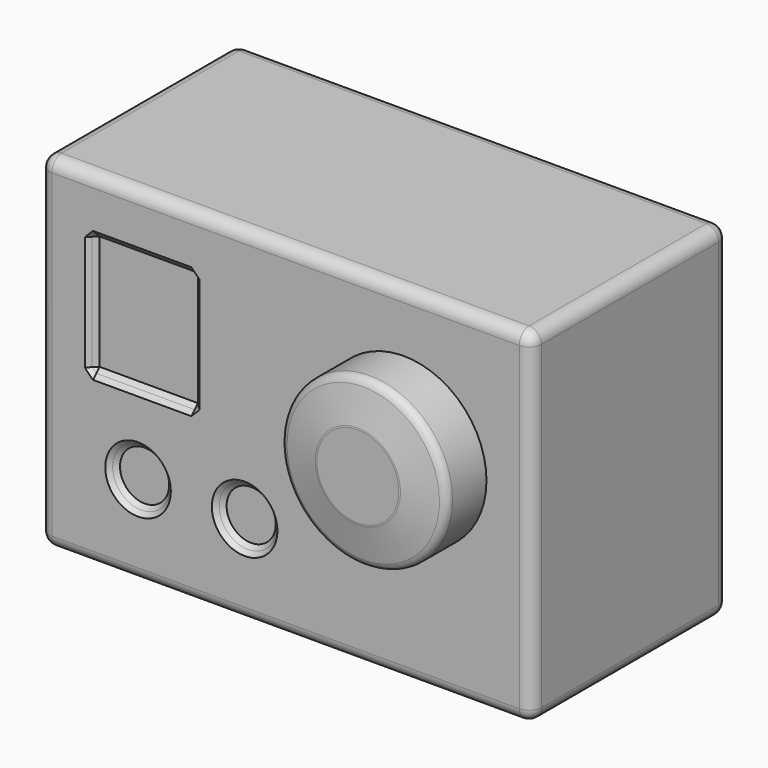
from build123d import *

# Parameters (mm, degrees)
F0_W     = 60
F0_H     = 42
F1_DEPTH = 30
F2_R     = 3.5
F2_W     = 13
F2_H     = 15
F3_DEPTH = 1
F4_SIZE  = 0.49999
F5_R     = 10.1
F6_DEPTH = 7
F7_SIZE2 = 1
F7_SIZE  = 5
F8_R     = 1
F9_R     = 1.5


# Not quite as in the source:
# - a fillet or chamfer is up to 0.001 mm smaller than in the source, because OpenCascade refuses the exact size


with BuildPart() as f1:
    # F0 (on Front) → F1 (new body)
    with BuildSketch(Plane.XZ):
        Rectangle(F0_W, F0_H)
    extrude(amount=F1_DEPTH)

    # F2 (on face) → F3 (cut)
    with BuildSketch(Plane.XZ.offset(30)):
        with Locations((-18, -10)):
            Circle(F2_R)
        with Locations((-5, -10)):
            Circle(F2_R)
        with Locations((-17.5, 6.9)):
            Rectangle(F2_W, F2_H)
    extrude(amount=-F3_DEPTH, mode=Mode.SUBTRACT)

    # F4 (size 0.5 in the source; OpenCascade refuses exactly that, so slightly less here)
    f4_edges = [f1.edges().sort_by_distance(p)[0] for p in [
        (-21.5, -30, -10),
        (-8.5, -30, -10),
        (-11, -30, 6.9),
        (-21.5, -29, -10),
        (-8.5, -29, -10),
        (-17.5, -30, 14.4),
        (-17.5, -30, -0.6),
        (-24, -30, 6.9),
        (-24, -29, 6.9),
        (-11, -29, 6.9),
        (-24, -29.5, 14.4),
        (-11, -29.5, 14.4),
        (-24, -29.5, -0.6),
        (-11, -29.5, -0.6),
        (-17.5, -29, 14.4),
        (-17.5, -29, -0.6),
    ]]
    chamfer(f4_edges, length=F4_SIZE)

    # F5 (on face) → F6 (join)
    with BuildSketch(Plane.XZ.offset(30)):
        with Locations((14.4, 3.7)):
            Circle(F5_R)
    extrude(amount=F6_DEPTH)

    # F7
    f7_edges = [f1.edges().sort_by_distance(p)[0] for p in [
        (4.3, -37, 3.7),
    ]]
    f7_side = f1.faces().sort_by_distance((14.4, -37, 3.7))[0]
    chamfer(f7_edges, length=F7_SIZE, length2=F7_SIZE2, reference=f7_side)

    # F8
    f8_edges = [f1.edges().sort_by_distance(p)[0] for p in [
        (9.3, -37, 3.7),
        (4.3, -36, 3.7),
    ]]
    fillet(f8_edges, radius=F8_R)

    # F9
    f9_edges = [f1.edges().sort_by_distance(p)[0] for p in [
        (30, -15, 21),
        (-30, -15, 21),
        (0, 0, 21),
        (0, -30, 21),
        (30, -15, -21),
        (30, 0, 0),
        (30, -30, 0),
        (-30, -15, -21),
        (0, 0, -21),
        (0, -30, -21),
        (-30, 0, 0),
        (-30, -30, 0),
    ]]
    fillet(f9_edges, radius=F9_R)


with BuildPart() as f10_1:
    # F10: copy of F1
    add(f1.part)


solid = Compound([f1.part, f10_1.part])
